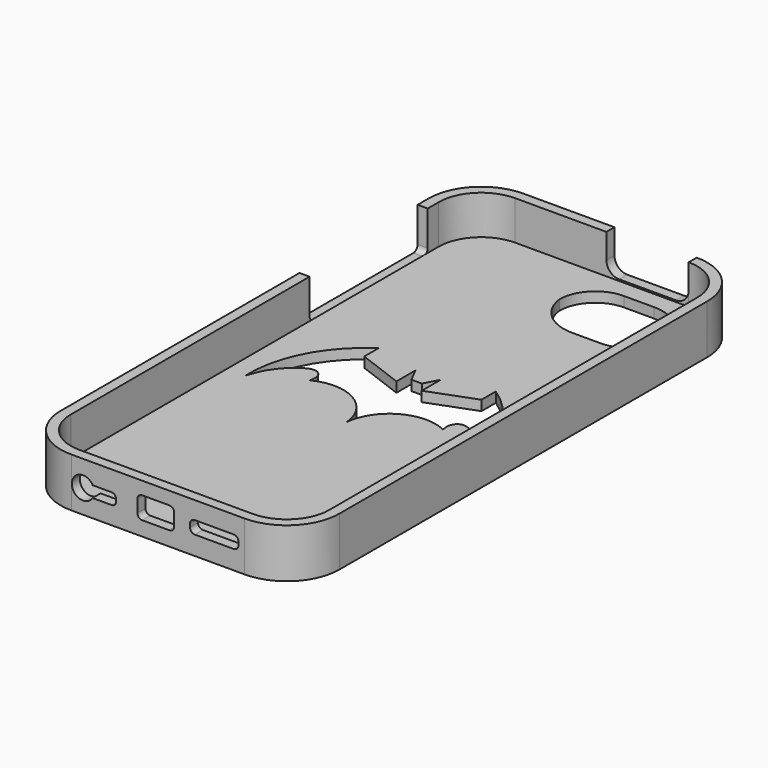
from build123d import *

# Parameters (mm, degrees)
F0_W         = 63.246
F0_H         = 128.27
F1_DEPTH     = 11.176
F2_R         = 11.938
F3_R         = 11.938
F4_R         = 11.938
F5_R         = 11.938
F6_T         = -2.286
F7_W         = 24.892
F7_H         = 16.764
F8_DEPTH     = 25.4
F9_R         = 8.128
F10_R        = 9.906
F11_R        = 8.128
F12_T1_DEPTH = 2.286
F13_W        = 2.286
F13_H        = 33.528
F14_DEPTH    = 9.144
F15_T1_DEPTH = 2.286
F16_T1_DEPTH = 2.286
F18_DEPTH    = 25.4
F19_R        = 1.016
F20_R        = 1.016
F21_W        = 8.3583914675
F21_H        = 4.9851476215
F22_DEPTH    = 25.4
F23_R        = 1.1037784407
F24_R        = 1.0922
F25_R        = 1.0922
F26_R        = 1.0922
F27_W        = 11.0163800418
F27_H        = 2.9015499167
F28_DEPTH    = 23.7236
F29_R        = 1.0922
F30_R        = 1.0922
F31_R        = 1.0922
F32_R        = 1.0922
F34_DEPTH    = 33.02
F35_W        = 18.6730868234
F35_H        = 2.286
F36_DEPTH    = 8.5344
F37_R        = 2.8820881508


# Not quite as in the source:
# - a fillet or chamfer that OpenCascade refuses, or shapes differently, is made with other operations: its cross-section is extruded or revolved along the edge and cut away or added


with BuildPart() as f1:
    # F0 (on Top) → F1 (new body)
    with BuildSketch(Plane.XY):
        Rectangle(F0_W, F0_H)
    extrude(amount=F1_DEPTH)

    # F2
    f2_edges = [f1.edges().sort_by_distance(p)[0] for p in [
        (-31.623, -64.135, 5.588),
    ]]
    fillet(f2_edges, radius=F2_R)

    # F3
    f3_edges = [f1.edges().sort_by_distance(p)[0] for p in [
        (31.623, -64.135, 5.588),
    ]]
    fillet(f3_edges, radius=F3_R)

    # F4
    f4_edges = [f1.edges().sort_by_distance(p)[0] for p in [
        (-31.623, 64.135, 5.588),
    ]]
    fillet(f4_edges, radius=F4_R)

    # F5
    f5_edges = [f1.edges().sort_by_distance(p)[0] for p in [
        (31.623, 64.135, 5.588),
    ]]
    fillet(f5_edges, radius=F5_R)

    # F6
    f6_openings = [f1.faces().sort_by_distance(p)[0] for p in [
        (0, 0, 11.176),
    ]]
    offset(amount=F6_T, openings=f6_openings)

    # F7 (on face) → F8 (cut)
    with BuildSketch(Plane(origin=(0, 0, 0), x_dir=(1, 0, 0), z_dir=(0, 0, -1))):
        with Locations((12.446, -49.521783433)):
            Rectangle(F7_W, F7_H)
    extrude(amount=-F8_DEPTH, mode=Mode.SUBTRACT)

    # F9
    f9_edges = [f1.edges().sort_by_distance(p)[0] for p in [
        (0, 57.903783, 1.143),
    ]]
    fillet(f9_edges, radius=F9_R)

    # F10
    f10_edges = [f1.edges().sort_by_distance(p)[0] for p in [
        (24.892, 57.903783, 1.143),
    ]]
    fillet(f10_edges, radius=F10_R)

    # F11
    f11_edges = [f1.edges().sort_by_distance(p)[0] for p in [
        (24.892, 41.139783, 1.143),
    ]]
    fillet(f11_edges, radius=F11_R)

    # F12: fillet of radius 9.906 on 1 edges, made by hand

    # F12_s2 → F12_t1 (join)
    with BuildSketch(Plane.XY):
        with BuildLine():
            ThreePointArc((9.8242524398, 41.139783433), (3.2840606994, 43.6057076269), (0, 49.775783433))
            Line((0, 49.775783433), (-0.1964850488, 49.750383433))
            ThreePointArc((-0.1964850488, 49.750383433), (-0.19812, 45.457783433), (-0.19812, 41.139783433))
            Line((-0.19812, 41.139783433), (0, 40.941663433))
            Line((0, 40.941663433), (9.8242524398, 40.941663433))
            Line((9.8242524398, 40.941663433), (9.8242524398, 41.139783433))
        make_face()
    extrude(amount=F12_T1_DEPTH)

    # F13 (on face) → F14 (cut)
    with BuildSketch(Plane.XY.offset(11.176)):
        with Locations((-30.48, 32.3110799655)):
            Rectangle(F13_W, F13_H)
    extrude(amount=-F14_DEPTH, mode=Mode.SUBTRACT)

    # F15: fillet of radius 1.2264204897 on 1 edges, made by hand

    # F15_s2 → F15_t1 (join)
    with BuildSketch(Plane.YZ.offset(-31.623)):
        with BuildLine():
            ThreePointArc((47.8486594758, 2.032), (48.7158697206, 2.3912102448), (49.0750799655, 3.2584204897))
            Line((49.0750799655, 3.2584204897), (49.0750799655, 2.032))
            Line((49.0750799655, 2.032), (47.8486594758, 2.032))
        make_face()
    extrude(amount=F15_T1_DEPTH)

    # F16: fillet of radius 1.2192 on 1 edges, made by hand

    # F16_s2 → F16_t1 (join)
    with BuildSketch(Plane.YZ.offset(-31.623)):
        with BuildLine():
            ThreePointArc((16.7662799655, 2.032), (15.9041753778, 2.3890954124), (15.5470799655, 3.2512))
            Line((15.5470799655, 3.2512), (15.5470799655, 2.032))
            Line((15.5470799655, 2.032), (16.7662799655, 2.032))
        make_face()
    extrude(amount=F16_T1_DEPTH)

    # F17 (on face) → F18 (cut)
    with BuildSketch(Plane.XZ.offset(64.135)):
        with BuildLine():
            Line((-9.4765355727, 6.6056444594), (-14.8105355727, 6.6056444594))
            ThreePointArc((-14.8105355727, 6.6056444594), (-19.5693630922, 5.4245616882), (-14.8652266091, 4.0416315305))
            Line((-14.8652266091, 4.0416315305), (-9.5312266091, 4.0416315305))
            Line((-9.5312266091, 4.0416315305), (-9.4765355727, 6.6056444594))
        make_face()
    extrude(amount=-F18_DEPTH, mode=Mode.SUBTRACT)

    # F19
    f19_edges = [f1.edges().sort_by_distance(p)[0] for p in [
        (-9.476536, -62.992, 6.605644),
    ]]
    fillet(f19_edges, radius=F19_R)

    # F20
    f20_edges = [f1.edges().sort_by_distance(p)[0] for p in [
        (-9.531227, -62.992, 4.041632),
    ]]
    fillet(f20_edges, radius=F20_R)

    # F21 (on face) → F22 (cut)
    with BuildSketch(Plane.XZ.offset(64.135)):
        with Locations((-0.4982303362, 5.7584403548)):
            Rectangle(F21_W, F21_H)
    extrude(amount=-F22_DEPTH, mode=Mode.SUBTRACT)

    # F23
    f23_edges = [f1.edges().sort_by_distance(p)[0] for p in [
        (-4.677426, -62.992, 3.265867),
    ]]
    fillet(f23_edges, radius=F23_R)

    # F24
    f24_edges = [f1.edges().sort_by_distance(p)[0] for p in [
        (3.680965, -62.992, 3.265867),
    ]]
    fillet(f24_edges, radius=F24_R)

    # F25
    f25_edges = [f1.edges().sort_by_distance(p)[0] for p in [
        (-4.677426, -62.992, 8.251014),
    ]]
    fillet(f25_edges, radius=F25_R)

    # F26
    f26_edges = [f1.edges().sort_by_distance(p)[0] for p in [
        (3.680965, -62.992, 8.251014),
    ]]
    fillet(f26_edges, radius=F26_R)

    # F27 (on face) → F28 (cut)
    with BuildSketch(Plane.XZ.offset(64.135)):
        with Locations((12.7713233232, 5.7310790289)):
            Rectangle(F27_W, F27_H)
    extrude(amount=-F28_DEPTH, mode=Mode.SUBTRACT)

    # F29
    f29_edges = [f1.edges().sort_by_distance(p)[0] for p in [
        (7.263133, -62.992, 7.181854),
    ]]
    fillet(f29_edges, radius=F29_R)

    # F30
    f30_edges = [f1.edges().sort_by_distance(p)[0] for p in [
        (7.263133, -62.992, 4.280304),
    ]]
    fillet(f30_edges, radius=F30_R)

    # F31
    f31_edges = [f1.edges().sort_by_distance(p)[0] for p in [
        (18.279513, -62.992, 7.181854),
    ]]
    fillet(f31_edges, radius=F31_R)

    # F32
    f32_edges = [f1.edges().sort_by_distance(p)[0] for p in [
        (18.279513, -62.992, 4.280304),
    ]]
    fillet(f32_edges, radius=F32_R)

    # F33 (on face) → F34 (cut)
    with BuildSketch(Plane(origin=(0, 0, 0), x_dir=(1, 0, 0), z_dir=(0, 0, -1))):
        with BuildLine():
            ThreePointArc((15.0896972045, 2.1444668528), (5.3363909856, 2.388488612), (0, 10.5560745509))
            Line((0, 10.5560745509), (0, -9.2810634524))
            Line((0, -9.2810634524), (1.1853649048, -9.2810634524))
            Line((1.1853649048, -9.2810634524), (2.8742128052, -12.5002330169))
            Line((2.8742128052, -12.5002330169), (2.8742128052, -7.1109388955))
            Line((2.8742128052, -7.1109388955), (13.3010493591, -11.026494205))
            Line((13.3010493591, -11.026494205), (13.3010493591, -15.0916064158))
            ThreePointArc((13.3010493591, -15.0916064158), (22.2319223209, -5.1790136532), (25.1711737365, 7.8356238082))
            add(Edge.make_bspline(
                [(15.0896972045, 2.1444668528), (14.9715152653, 1.4144964774), (14.7345248911, -0.0493139285), (16.7022230876, -2.1698757875), (20.3604436705, -0.0674466541), (22.2531707468, 2.0801196366), (24.023585933, 4.5420730619), (24.7774674064, 6.7056956465), (25.1711737365, 7.8356238082)],
                knots=[0, 0, 0, 0, 0.1438529036, 0.2884683875, 0.4775038189, 0.6479653876, 0.8161537852, 1, 1, 1, 1], degree=3))
        make_face()
        with BuildLine():
            Line((0, -9.2810634524), (0, 10.5560745509))
            ThreePointArc((0, 10.5560745509), (-5.3363909856, 2.388488612), (-15.0896972045, 2.1444668528))
            add(Edge.make_bspline(
                [(-15.0896972045, 2.1444668528), (-14.9715152653, 1.4144964774), (-14.7345248911, -0.0493139285), (-16.7022230876, -2.1698757875), (-20.3604436705, -0.0674466541), (-22.2531707468, 2.0801196366), (-24.023585933, 4.5420730619), (-24.7774674064, 6.7056956465), (-25.1711737365, 7.8356238082)],
                knots=[0, 0, 0, 0, 0.1438529036, 0.2884683875, 0.4775038189, 0.6479653876, 0.8161537852, 1, 1, 1, 1], degree=3))
            ThreePointArc((-25.1711737365, 7.8356238082), (-22.2319223209, -5.1790136532), (-13.3010493591, -15.0916064158))
            Line((-13.3010493591, -15.0916064158), (-13.3010493591, -11.026494205))
            Line((-13.3010493591, -11.026494205), (-2.8742128052, -7.1109388955))
            Line((-2.8742128052, -7.1109388955), (-2.8742128052, -12.5002330169))
            Line((-2.8742128052, -12.5002330169), (-1.1853649048, -9.2810634524))
            Line((-1.1853649048, -9.2810634524), (0, -9.2810634524))
        make_face()
    extrude(amount=-F34_DEPTH, mode=Mode.SUBTRACT)

    # F35 (on face) → F36 (cut)
    with BuildSketch(Plane.XY.offset(11.176)):
        with Locations((10.3484565883, 62.992)):
            Rectangle(F35_W, F35_H)
    extrude(amount=-F36_DEPTH, mode=Mode.SUBTRACT)

    # F37
    f37_edges = [f1.edges().sort_by_distance(p)[0] for p in [
        (19.685, 62.992, 2.6416),
        (1.011913, 62.992, 2.6416),
    ]]
    fillet(f37_edges, radius=F37_R)


solid = f1.part
